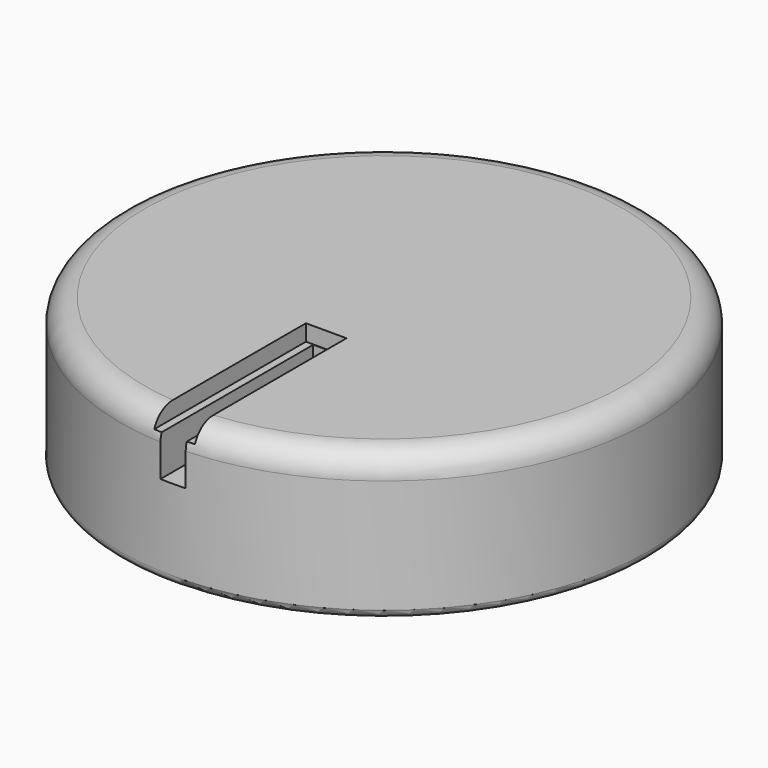
from build123d import *

# Parameters (mm, degrees)
F0_R      = 32.5
F1_DEPTH  = 18
F2_R      = 3
F3_R      = 1
F4_R      = 25.405
F5_DEPTH  = 9.104
F6_R      = 27.5
F6_R_2    = 25.405
F7_DEPTH  = 1.5
F9_DEPTH  = 7
F11_DEPTH = 2


# Not quite as in the source:
# - the program builds the solid bodies; features that only make, move or delete a surface that nothing else refers to are left out


with BuildPart() as f1:
    # F0 (on Top) → F1 (new body)
    with BuildSketch(Plane.XY):
        Circle(F0_R)
    extrude(amount=F1_DEPTH)

    # F2
    f2_edges = [f1.edges().sort_by_distance(p)[0] for p in [
        (-32.5, 0, 18),
    ]]
    fillet(f2_edges, radius=F2_R)

    # F3
    f3_edges = [f1.edges().sort_by_distance(p)[0] for p in [
        (-32.5, 0, 0),
    ]]
    fillet(f3_edges, radius=F3_R)

    # F4 (on face) → F5 (cut)
    with BuildSketch(Plane(origin=(0, 0, 0), x_dir=(1, 0, 0), z_dir=(0, 0, -1))):
        Circle(F4_R)
    extrude(amount=-F5_DEPTH, mode=Mode.SUBTRACT)

    # F6 (on face) → F7 (cut)
    with BuildSketch(Plane(origin=(0, 0, 0), x_dir=(1, 0, 0), z_dir=(0, 0, -1))):
        Circle(F6_R)
        Circle(F6_R_2, mode=Mode.SUBTRACT)
    extrude(amount=-F7_DEPTH, mode=Mode.SUBTRACT)

    # F8 (on face) → F9 (cut)
    with BuildSketch(Plane.XY.offset(18)):
        with BuildLine():
            Line((1.55, -8.9630174198), (0, -8.9630174198))
            Line((0, -8.9630174198), (-1.55, -8.9630174198))
            Line((-1.55, -8.9630174198), (-1.55, -29.459251518))
            ThreePointArc((-1.55, -29.459251518), (0, -29.5), (1.55, -29.459251518))
            Line((1.55, -29.459251518), (1.55, -8.9630174198))
        make_face()
        with BuildLine():
            Line((1.55, -32.4630174198), (1.55, -29.459251518))
            ThreePointArc((1.55, -29.459251518), (0, -29.5), (-1.55, -29.459251518))
            Line((-1.55, -29.459251518), (-1.55, -32.4630174198))
            ThreePointArc((-1.55, -32.4630174198), (0, -32.5), (1.55, -32.4630174198))
        make_face()
    extrude(amount=-F9_DEPTH, mode=Mode.SUBTRACT)

    # F10 (on face) → F11 (cut)
    with BuildSketch(Plane.XY.offset(18)):
        with BuildLine():
            ThreePointArc((-2.5, -32.403703492), (-2.0252171576, -32.4368385553), (-1.55, -32.4630174198))
            ThreePointArc((-1.55, -32.4630174198), (0, -32.5), (1.55, -32.4630174198))
            ThreePointArc((1.55, -32.4630174198), (2.0252171576, -32.4368385553), (2.5, -32.403703492))
            Line((2.5, -32.403703492), (2.5, -8.903703492))
            Line((2.5, -8.903703492), (-2.5, -8.903703492))
            Line((-2.5, -8.903703492), (-2.5, -32.403703492))
        make_face()
    extrude(amount=-F11_DEPTH, mode=Mode.SUBTRACT)


solid = f1.part
